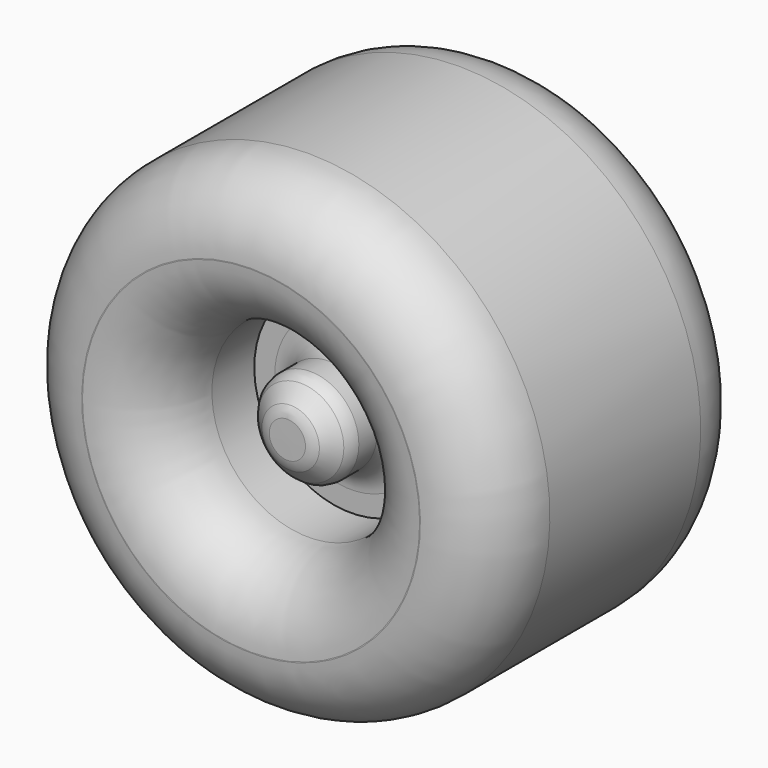
from build123d import *

# Parameters (mm, degrees)
F0_W   = 44.9125468731
F0_H   = 37.5907570124
F0_W_2 = 45.6432104111
F4_R   = 55.8969601189
F5_R   = 12.5522501698
F6_R   = 21.6676277208


with BuildPart() as f2:
    # F1 (on face) → F2 (revolve)
    with BuildSketch(Plane.YZ):
        Polygon((130.2607655525, 75.1815140247), (130.2607655525, 187.6416653395), (-128.1981468201, 187.6416653395), (-128.1981468201, 75.1815140247), (-31.1205983162, 75.1815140247), (29.1936397552, 75.1815140247), align=None)
    revolve(axis=Axis((0, -0.9634792805, 0), (0, 1, 0)))

    # F4
    f4_edges = [f2.edges().sort_by_distance(p)[0] for p in [
        (0, -128.198147, -187.641665),
        (0, 130.260766, -187.641665),
        (0, 130.260766, -75.181514),
        (0, -128.198147, -75.181514),
    ]]
    fillet(f4_edges, radius=F4_R)


with BuildPart() as f3:
    # F0 (on Right) → F3 (revolve)
    with BuildSketch(Plane.YZ):
        Polygon((29.1936397552, 75.1815140247), (-31.1205983162, 75.1815140247), (-31.1205983162, 37.5907570124), (-31.1205983162, 0), (29.1936397552, 0), (29.1936397552, 37.5907570124), align=None)
        with Locations((-53.5768717527, 18.7953785062)):
            Rectangle(F0_W, F0_H)
        Polygon((-76.0331451893, 0), (-76.0331451893, 37.5907570124), (-92.8205251694, 18.7953785062), (-92.9662585258, 0), align=None)
        with Locations((52.0152449608, 18.7953785062)):
            Rectangle(F0_W_2, F0_H)
        Polygon((96.821308136, 18.7953785062), (74.8368501663, 37.5907570124), (74.8368501663, 0), (96.821308136, 0), align=None)
    revolve(axis=Axis((0, -0.9634792805, 0), (0, 1, 0)))

    # F5
    f5_edges = [f3.edges().sort_by_distance(p)[0] for p in [
        (0, -76.033145, -37.590757),
        (0, -92.820525, -18.795379),
        (0, 74.83685, -37.590757),
        (0, 96.821308, -18.795379),
    ]]
    fillet(f5_edges, radius=F5_R)

    # F6
    f6_edges = [f3.edges().sort_by_distance(p)[0] for p in [
        (0, -31.120598, -37.590757),
        (0, 29.19364, -37.590757),
    ]]
    fillet(f6_edges, radius=F6_R)


solid = Compound([f2.part, f3.part])
